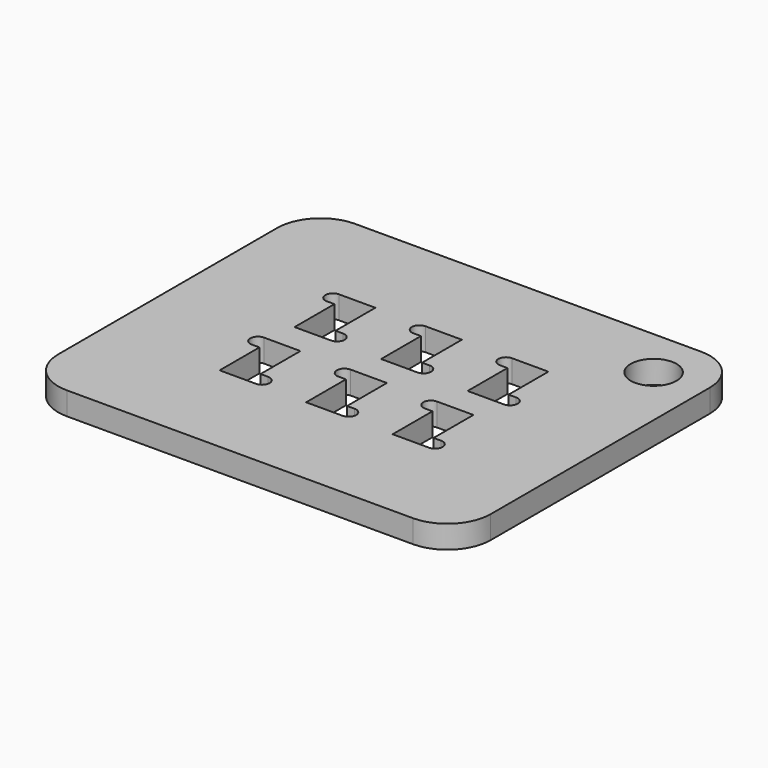
from build123d import *

# Parameters (mm, degrees)
F0_R     = 1.5875
F1_DEPTH = 1.5875


# Not quite as in the source:
# - a length typed as a fraction of an inch, garbled in the dataset ("3 / 203.2 mm" for 3/8 in), is restored


with BuildPart() as f1:
    # F0 (on Top) → F1 (new body)
    with BuildSketch(Plane.XY):
        with BuildLine():
            Line((-6, -12.5), (18, -12.5))
            ThreePointArc((18, -12.5), (20.1213203436, -11.6213203436), (21, -9.5))
            Line((21, -9.5), (21, 9.5))
            ThreePointArc((21, 9.5), (20.1213203436, 11.6213203436), (18, 12.5))
            Line((18, 12.5), (-6, 12.5))
            ThreePointArc((-6, 12.5), (-8.1213203436, 11.6213203436), (-9, 9.5))
            Line((-9, 9.5), (-9, -9.5))
            ThreePointArc((-9, -9.5), (-8.1213203436, -11.6213203436), (-6, -12.5))
        make_face()
        with BuildLine():
            Line((1.525, -5.5), (1, -5.5))
            Line((1, -5.5), (-1, -5.5))
            Line((-1, -5.5), (-1, -2.05))
            Line((-1, -2.05), (-1.525, -2.05))
            ThreePointArc((-1.525, -2.05), (-2.05, -1.525), (-1.525, -1))
            Line((-1.525, -1), (-1, -1))
            Line((-1, -1), (1, -1))
            Line((1, -1), (1, -4.45))
            Line((1, -4.45), (1.525, -4.45))
            ThreePointArc((1.525, -4.45), (2.05, -4.975), (1.525, -5.5))
        make_face(mode=Mode.SUBTRACT)
        with BuildLine():
            Line((7.525, -5.5), (7, -5.5))
            Line((7, -5.5), (5, -5.5))
            Line((5, -5.5), (5, -2.05))
            Line((5, -2.05), (4.475, -2.05))
            ThreePointArc((4.475, -2.05), (3.95, -1.525), (4.475, -1))
            Line((4.475, -1), (5, -1))
            Line((5, -1), (7, -1))
            Line((7, -1), (7, -4.45))
            Line((7, -4.45), (7.525, -4.45))
            ThreePointArc((7.525, -4.45), (8.05, -4.975), (7.525, -5.5))
        make_face(mode=Mode.SUBTRACT)
        with BuildLine():
            Line((13.525, -5.5), (13, -5.5))
            Line((13, -5.5), (11, -5.5))
            Line((11, -5.5), (11, -2.05))
            Line((11, -2.05), (10.475, -2.05))
            ThreePointArc((10.475, -2.05), (9.95, -1.525), (10.475, -1))
            Line((10.475, -1), (11, -1))
            Line((11, -1), (13, -1))
            Line((13, -1), (13, -4.45))
            Line((13, -4.45), (13.525, -4.45))
            ThreePointArc((13.525, -4.45), (14.05, -4.975), (13.525, -5.5))
        make_face(mode=Mode.SUBTRACT)
        with BuildLine():
            Line((-1, 5.5), (1, 5.5))
            Line((1, 5.5), (1, 2.05))
            Line((1, 2.05), (1.525, 2.05))
            ThreePointArc((1.525, 2.05), (2.05, 1.525), (1.525, 1))
            Line((1.525, 1), (1, 1))
            Line((1, 1), (-1, 1))
            Line((-1, 1), (-1, 4.45))
            Line((-1, 4.45), (-1.525, 4.45))
            ThreePointArc((-1.525, 4.45), (-2.05, 4.975), (-1.525, 5.5))
            Line((-1.525, 5.5), (-1, 5.5))
        make_face(mode=Mode.SUBTRACT)
        with BuildLine():
            Line((7.525, 1), (7, 1))
            Line((7, 1), (5, 1))
            Line((5, 1), (5, 4.45))
            Line((5, 4.45), (4.475, 4.45))
            ThreePointArc((4.475, 4.45), (3.95, 4.975), (4.475, 5.5))
            Line((4.475, 5.5), (5, 5.5))
            Line((5, 5.5), (7, 5.5))
            Line((7, 5.5), (7, 2.05))
            Line((7, 2.05), (7.525, 2.05))
            ThreePointArc((7.525, 2.05), (8.05, 1.525), (7.525, 1))
        make_face(mode=Mode.SUBTRACT)
        with BuildLine():
            Line((13.525, 1), (13, 1))
            Line((13, 1), (11, 1))
            Line((11, 1), (11, 4.45))
            Line((11, 4.45), (10.475, 4.45))
            ThreePointArc((10.475, 4.45), (9.95, 4.975), (10.475, 5.5))
            Line((10.475, 5.5), (11, 5.5))
            Line((11, 5.5), (13, 5.5))
            Line((13, 5.5), (13, 2.05))
            Line((13, 2.05), (13.525, 2.05))
            ThreePointArc((13.525, 2.05), (14.05, 1.525), (13.525, 1))
        make_face(mode=Mode.SUBTRACT)
        with Locations((17.5, 9)):
            Circle(F0_R, mode=Mode.SUBTRACT)
    extrude(amount=F1_DEPTH)


solid = f1.part
